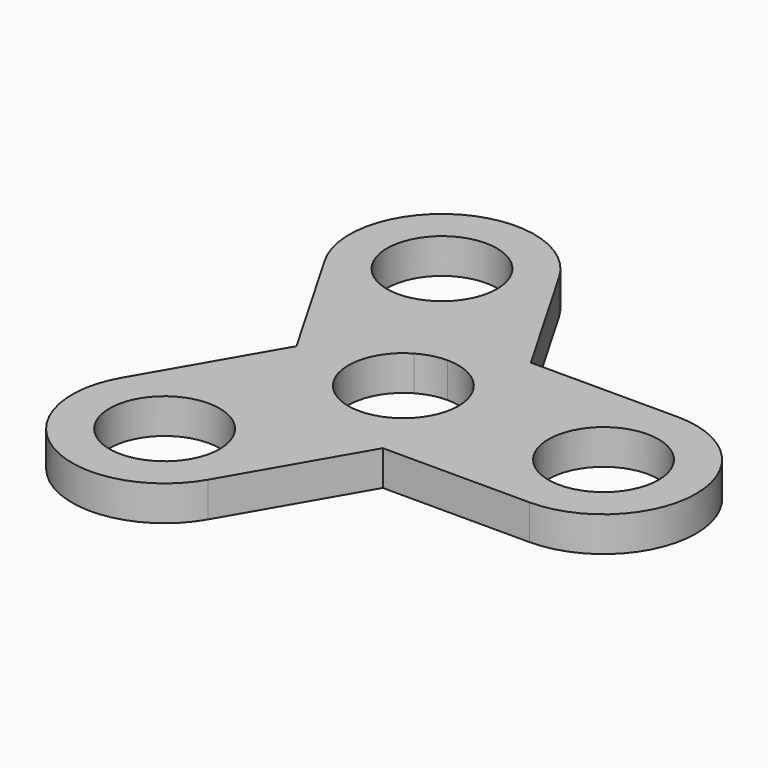
from build123d import *

# Parameters (mm, degrees)
F0_R            = 11
F1_DEPTH        = 7
F1_COPIES_COUNT = 3


# Not quite as in the source:
# - a pattern or mirror of a feature is missing from the dataset's text; its kind, count and spacing are read off the source's solid


with BuildPart() as f1:
    # F0 (on Top) → F1 (new body)
    with BuildSketch(Plane.XY):
        with BuildLine():
            ThreePointArc((0, 11), (7.7781745931, 7.7781745931), (11, 0))
            ThreePointArc((11, 0), (7.7781745931, -7.7781745931), (0, -11))
            Line((0, -11), (0, -18.5))
            Line((0, -18.5), (40, -18.5))
            ThreePointArc((40, -18.5), (58.5, 0), (40, 18.5))
            Line((40, 18.5), (0, 18.5))
            Line((0, 18.5), (0, 11))
        make_face()
        with Locations((40, 0)):
            Circle(F0_R, mode=Mode.SUBTRACT)
    extrude(amount=F1_DEPTH)

    # F1_copies: F1 ×3 about axis
    f1_copies_axis = Axis((0, 0, 0), (0, 0, 1))


with BuildPart() as f1_1:
    add(f1.part)
    for i in range(1, F1_COPIES_COUNT):
        add(f1.part.rotate(f1_copies_axis, i * 360 / F1_COPIES_COUNT))


solid = f1_1.part
